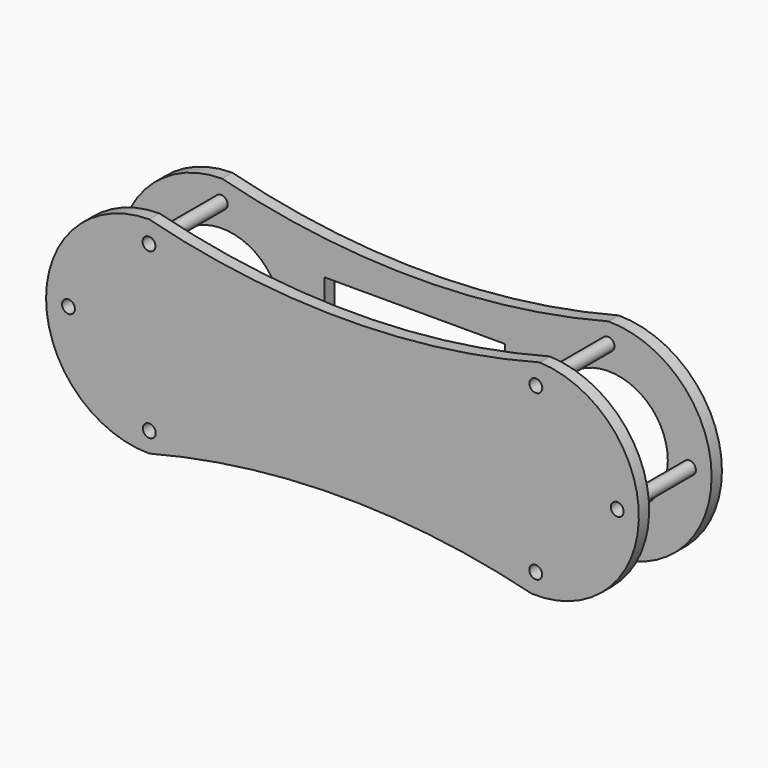
from build123d import *

# Parameters (mm, degrees)
F0_R     = 23
F0_W     = 70
F0_H     = 38
F1_DEPTH = 5
F3_R     = 2.5
F4_DEPTH = 5
F5_DEPTH = 30


with BuildPart() as f1:
    # F0 (on Front) → F1 (new body)
    with BuildSketch(Plane.XZ):
        with BuildLine():
            ThreePointArc((-74.7628004057, -40.2371987939), (0.2371995943, -30.7109497595), (75.2371995943, -40.2371987939))
            ThreePointArc((75.2371995943, -40.2371987939), (115.2371995943, -0.2371987939), (75.2371995943, 39.7628012061))
            ThreePointArc((75.2371995943, 39.7628012061), (0.2371995943, 30.2365521716), (-74.7628004057, 39.7628012061))
            ThreePointArc((-74.7628004057, 39.7628012061), (-114.7628004057, -0.2371987939), (-74.7628004057, -40.2371987939))
        make_face()
        with Locations((75.2371995943, -0.2371987939)):
            Circle(F0_R, mode=Mode.SUBTRACT)
        with Locations((-74.7628004057, -0.2371987939)):
            Circle(F0_R, mode=Mode.SUBTRACT)
        Rectangle(F0_W, F0_H, mode=Mode.SUBTRACT)
    extrude(amount=F1_DEPTH)


with BuildPart() as f4:
    # F3 (on offset) → F4 (new body)
    with BuildSketch(Plane.XZ.offset(35)):
        with BuildLine():
            ThreePointArc((-75.0000307412, -40.0000089742), (-0.8211479846, -30.4748836644), (73.4087647878, -39.593804049))
            ThreePointArc((73.4087647878, -39.593804049), (114.9823591797, -1.1673984409), (76.5559535716, 40.406195951))
            ThreePointArc((76.5559535716, 40.406195951), (0.8040354288, 30.4748195307), (-75.0000307412, 39.9999910258))
            ThreePointArc((-75.0000307412, 39.9999910258), (-115.0000307412, -8.9742e-06), (-75.0000307412, -40.0000089742))
        make_face()
        with Locations((-74.9454423785, -32.203219831)):
            Circle(F3_R, mode=Mode.SUBTRACT)
        with Locations((-106.3136458397, 0)):
            Circle(F3_R, mode=Mode.SUBTRACT)
        with Locations((74.9903470278, -31.7338556051)):
            Circle(F3_R, mode=Mode.SUBTRACT)
        with Locations((106.6243350506, 0)):
            Circle(F3_R, mode=Mode.SUBTRACT)
        with Locations((-75.0656053424, 31.6041447222)):
            Circle(F3_R, mode=Mode.SUBTRACT)
        with Locations((75.0285089016, 31.9726653397)):
            Circle(F3_R, mode=Mode.SUBTRACT)
    extrude(amount=F4_DEPTH)


with BuildPart() as f5:
    # F3 (on offset) → F5 (new body)
    with BuildSketch(Plane.XZ.offset(35)):
        with Locations((-75.0656053424, 31.6041447222)):
            Circle(F3_R)
    extrude(amount=-F5_DEPTH)


with BuildPart() as f5b:
    # F3 (on offset) → F5, piece 2 (new body)
    with BuildSketch(Plane.XZ.offset(35)):
        with Locations((-106.3136458397, 0)):
            Circle(F3_R)
    extrude(amount=-F5_DEPTH)


with BuildPart() as f5c:
    # F3 (on offset) → F5, piece 3 (new body)
    with BuildSketch(Plane.XZ.offset(35)):
        with Locations((-74.9454423785, -32.203219831)):
            Circle(F3_R)
    extrude(amount=-F5_DEPTH)


with BuildPart() as f5d:
    # F3 (on offset) → F5, piece 4 (new body)
    with BuildSketch(Plane.XZ.offset(35)):
        with Locations((75.0285089016, 31.9726653397)):
            Circle(F3_R)
    extrude(amount=-F5_DEPTH)


with BuildPart() as f5e:
    # F3 (on offset) → F5, piece 5 (new body)
    with BuildSketch(Plane.XZ.offset(35)):
        with Locations((106.6243350506, 0)):
            Circle(F3_R)
    extrude(amount=-F5_DEPTH)


with BuildPart() as f5f:
    # F3 (on offset) → F5, piece 6 (new body)
    with BuildSketch(Plane.XZ.offset(35)):
        with Locations((74.9903470278, -31.7338556051)):
            Circle(F3_R)
    extrude(amount=-F5_DEPTH)


solid = Compound([f1.part, f4.part, f5.part, f5b.part, f5c.part, f5d.part, f5e.part, f5f.part])
